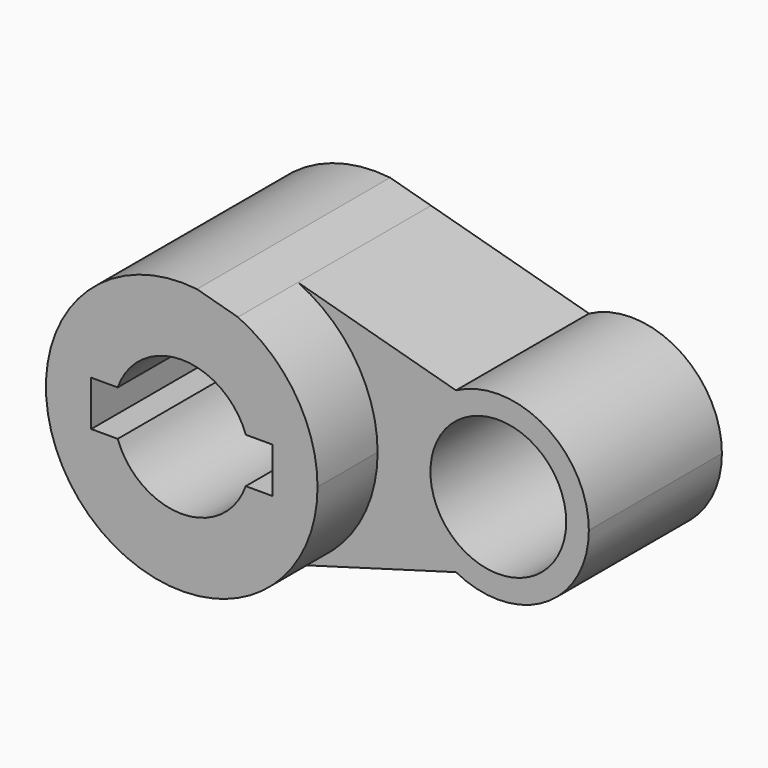
from build123d import *

# Parameters (mm, degrees)
F0_R     = 14.2875
F1_DEPTH = 35
F2_DEPTH = 50.8


with BuildPart() as f1:
    # F0 (on Front) → F1 (new body)
    with BuildSketch(Plane.XZ):
        with BuildLine():
            Line((11.8201890877, 26.0156444266), (3.2047751505, 28.3947185447))
            ThreePointArc((3.2047751505, 28.3947185447), (-28.5220001461, -1.739578301), (6.631814894, -27.7947774989))
            Line((6.631814894, -27.7947774989), (9.0167764908, -27.1150948129))
            ThreePointArc((9.0167764908, -27.1150948129), (23.1752563441, -16.7164026748), (28.575, 0))
            ThreePointArc((28.575, 0), (24.0238686329, 15.47205096), (11.8201890877, 26.0156444266))
        make_face()
        with BuildLine():
            ThreePointArc((-13.4703841816, 4.7625), (0, 14.2875), (13.4703841816, 4.7625))
            Line((13.4703841816, 4.7625), (19.05, 4.7625))
            Line((19.05, 4.7625), (19.05, -4.7625))
            Line((19.05, -4.7625), (13.4703841816, -4.7625))
            ThreePointArc((13.4703841816, -4.7625), (0, -14.2875), (-13.4703841816, -4.7625))
            Line((-13.4703841816, -4.7625), (-19.05, -4.7625))
            Line((-19.05, -4.7625), (-19.05, 4.7625))
            Line((-19.05, 4.7625), (-13.4703841816, 4.7625))
        make_face(mode=Mode.SUBTRACT)
        with BuildLine():
            Line((45.0618756476, 16.8362321877), (11.8201890877, 26.0156444266))
            ThreePointArc((11.8201890877, 26.0156444266), (24.0238686329, 15.47205096), (28.575, 0))
            ThreePointArc((28.575, 0), (23.1752563441, -16.7164026748), (9.0167764908, -27.1150948129))
            Line((9.0167764908, -27.1150948129), (45.0698397536, -16.8404459854))
            ThreePointArc((45.0698397536, -16.8404459854), (34.9250005327, -0.0045050825), (45.0618756476, 16.8362321877))
        make_face()
        with BuildLine():
            ThreePointArc((73.025, 0), (63.8011762931, 16.3201948351), (45.0618756476, 16.8362321877))
            ThreePointArc((45.0618756476, 16.8362321877), (34.9250005327, -0.0045050825), (45.0698397536, -16.8404459854))
            ThreePointArc((45.0698397536, -16.8404459854), (63.8050355367, -16.3178706131), (73.025, 0))
        make_face()
        with Locations((53.975, 0)):
            Circle(F0_R, mode=Mode.SUBTRACT)
    extrude(amount=F1_DEPTH)

    # F0 (on Front) → F2 (join)
    with BuildSketch(Plane.XZ):
        with BuildLine():
            Line((11.8201890877, 26.0156444266), (3.2047751505, 28.3947185447))
            ThreePointArc((3.2047751505, 28.3947185447), (-28.5220001461, -1.739578301), (6.631814894, -27.7947774989))
            Line((6.631814894, -27.7947774989), (9.0167764908, -27.1150948129))
            ThreePointArc((9.0167764908, -27.1150948129), (23.1752563441, -16.7164026748), (28.575, 0))
            ThreePointArc((28.575, 0), (24.0238686329, 15.47205096), (11.8201890877, 26.0156444266))
        make_face()
        with BuildLine():
            ThreePointArc((-13.4703841816, 4.7625), (0, 14.2875), (13.4703841816, 4.7625))
            Line((13.4703841816, 4.7625), (19.05, 4.7625))
            Line((19.05, 4.7625), (19.05, -4.7625))
            Line((19.05, -4.7625), (13.4703841816, -4.7625))
            ThreePointArc((13.4703841816, -4.7625), (0, -14.2875), (-13.4703841816, -4.7625))
            Line((-13.4703841816, -4.7625), (-19.05, -4.7625))
            Line((-19.05, -4.7625), (-19.05, 4.7625))
            Line((-19.05, 4.7625), (-13.4703841816, 4.7625))
        make_face(mode=Mode.SUBTRACT)
    extrude(amount=F2_DEPTH)


solid = f1.part
